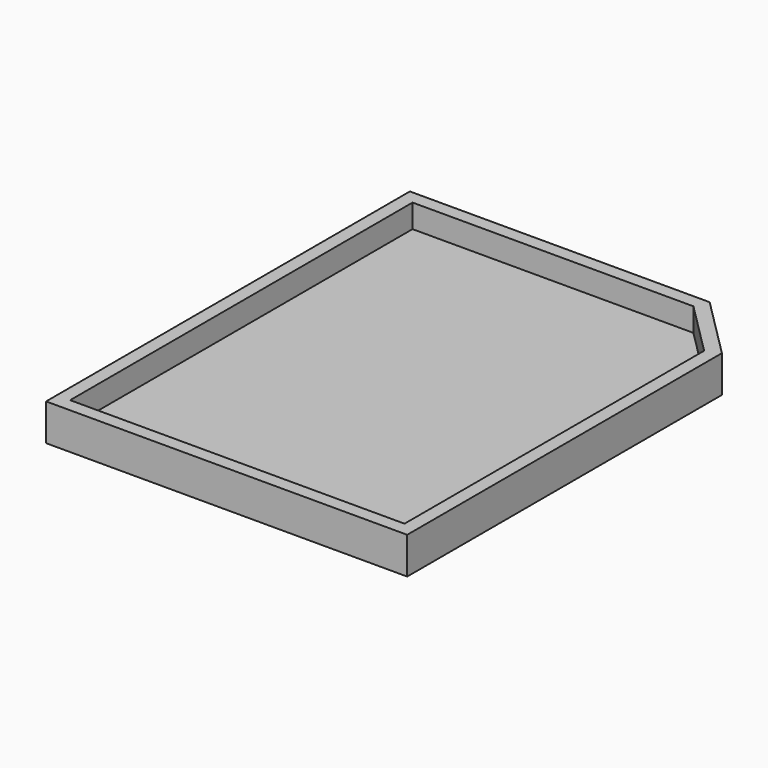
from build123d import *

# Parameters (mm, degrees)
F1_DEPTH = 1.75
F2_T     = 1


with BuildPart() as f1:
    # F0 (on Top) → F1 (new body)
    with BuildSketch(Plane.XY):
        Polygon((39.8734986782, 16), (39.8734986782, -16), (64.8734986782, -16), (64.8734986782, 12), (60.8734986782, 16), align=None)
    extrude(amount=F1_DEPTH)

    # F2
    f2_openings = [f1.faces().sort_by_distance(p)[0] for p in [
        (52.260704, -0.148148, 1.75),
    ]]
    offset(amount=F2_T, openings=f2_openings, kind=Kind.INTERSECTION)


solid = f1.part
